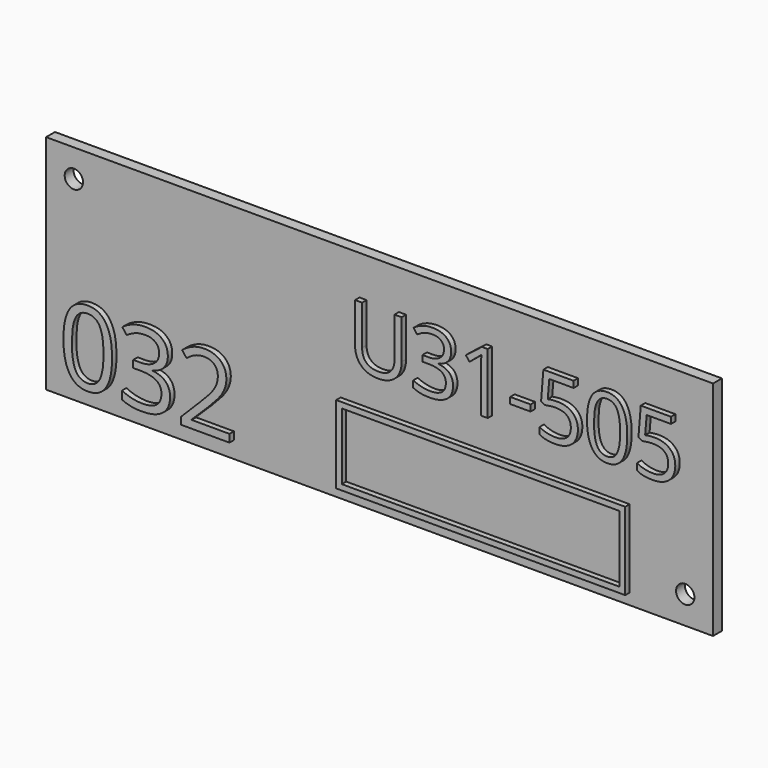
from build123d import *

# Parameters (mm, degrees)
F0_W         = 120
F0_H         = 40
F1_DEPTH     = 2
F3_D         = 3.3
F4_TEXT_SIZE = 15.3232242618
F5_DEPTH     = 1
F6_TEXT_SIZE = 18.5356140827
F7_DEPTH     = 1
F8_W         = 52
F8_H         = 14
F8_W_2       = 49.99999962
F8_H_2       = 11.99999962
F9_DEPTH     = 1


# Not quite as in the source:
# - Text() gives the source's letters only with a copy of the font that has no kerning and outlines rounded to 1/6400 em; it was checked with that copy


with BuildPart() as f1:
    # F0 (on Front) → F1 (new body)
    with BuildSketch(Plane.XZ):
        Rectangle(F0_W, F0_H)
    extrude(amount=F1_DEPTH)

    # F3 (through all)
    with Locations(Plane.XZ.offset(2)):
        with Locations((-55, 15), (55, -15)):
            Hole(F3_D / 2)

    # F4 (on face) → F5 (join)
    with BuildSketch(Plane.XZ.offset(2)):
        with Locations((-5, 2)):
            Text('U31-505', F4_TEXT_SIZE, font='Open Sans', text_align=(TextAlign.LEFT, TextAlign.BOTTOM))
    extrude(amount=F5_DEPTH)

    # F6 (on face) → F7 (join)
    with BuildSketch(Plane.XZ.offset(2)):
        with Locations((-57, -17)):
            Text('032', F6_TEXT_SIZE, font='Open Sans', text_align=(TextAlign.LEFT, TextAlign.BOTTOM))
    extrude(amount=F7_DEPTH)

    # F8 (on face) → F9 (join)
    with BuildSketch(Plane.XZ.offset(2)):
        with Locations((19, -11)):
            Rectangle(F8_W, F8_H)
        with Locations((19, -11)):
            Rectangle(F8_W_2, F8_H_2, mode=Mode.SUBTRACT)
    extrude(amount=F9_DEPTH)


solid = f1.part
